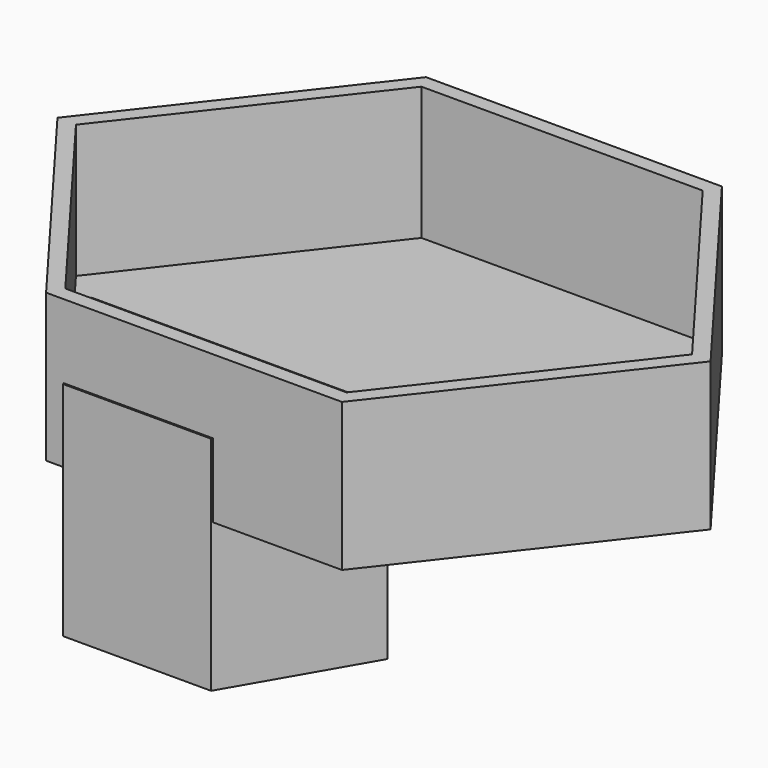
from build123d import *

# Parameters (mm, degrees)
F1_DEPTH      = 25.4
F2_T          = -2.54
F8_DEPTH      = 12.7
F8_DEPTH_BACK = 25.4


# Not quite as in the source:
# - the program builds the solid bodies; features that only make, move or delete a surface that nothing else refers to are left out


with BuildPart() as f1:
    # F0 (on Top) → F1 (new body)
    with BuildSketch(Plane.XY):
        Polygon((10.2551429075, 58.9377772835), (-40.5448570925, 58.9377772835), (-71.7704754875, 18.8678289949), (-41.2404706852, -21.7346192906), (9.5595293148, -21.7346192906), (40.7851477097, 18.335328998), align=None)
    extrude(amount=F1_DEPTH)

    # F2
    f2_openings = [f1.faces().sort_by_distance(p)[0] for p in [
        (-15.492664, 18.601579, 25.4),
    ]]
    offset(amount=F2_T, openings=f2_openings)

    # F7 (on Top) → F8 (join, two sides)
    with BuildSketch(Plane.XY) as f8_sk:
        Polygon((0, 0), (-50.8, 0), (-38.1, -21.9970452561), (-12.7, -21.9970452561), align=None)
    extrude(amount=F8_DEPTH)
    extrude(f8_sk.sketch, amount=-F8_DEPTH_BACK)


solid = f1.part
